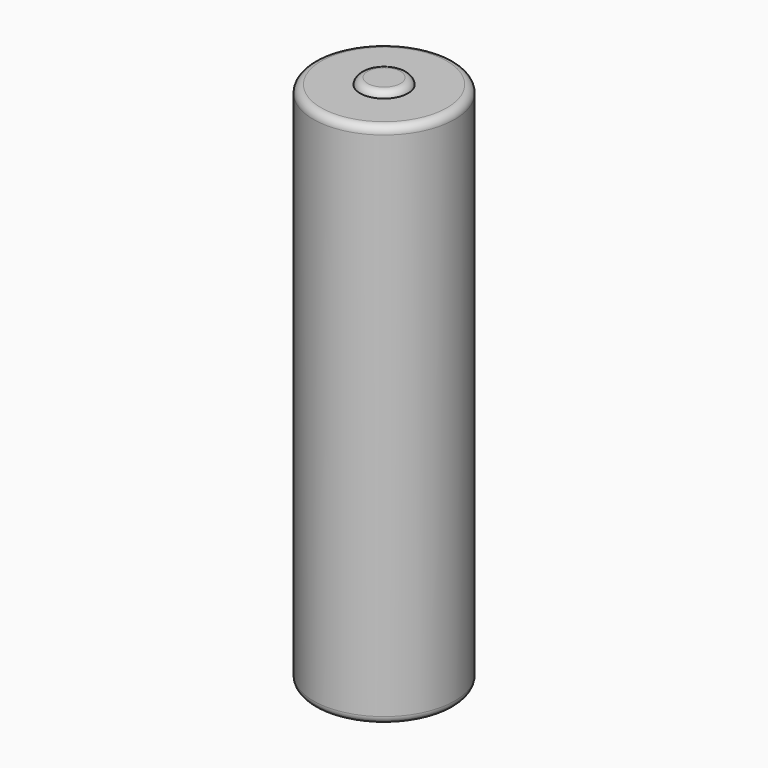
from build123d import *

# Parameters (mm, degrees)
F0_R     = 9.15
F0_R_2   = 3.1
F1_DEPTH = 68.2
F2_DEPTH = 69


# Not quite as in the source:
# - a fillet or chamfer that OpenCascade refuses, or shapes differently, is made with other operations: its cross-section is extruded or revolved along the edge and cut away or added


with BuildPart() as f1:
    # F0 (on Top) → F1 (new body)
    with BuildSketch(Plane.XY):
        Circle(F0_R)
        Circle(F0_R_2, mode=Mode.SUBTRACT)
    extrude(amount=F1_DEPTH)

    # F0 (on Top) → F2 (join)
    with BuildSketch(Plane.XY):
        Circle(F0_R_2)
    extrude(amount=F2_DEPTH)

    # F3: fillet of radius 1 on 3 edges, made by hand

    # F3_s1 → F3_t2 (revolve, cut)
    with BuildSketch(Plane.XZ):
        with BuildLine():
            ThreePointArc((3.1, 68.2), (2.7526596349, 68.7745966692), (2.1202041029, 69))
            Line((2.1202041029, 69), (3.1, 69))
            Line((3.1, 69), (3.1, 68.2))
        make_face()
    revolve(axis=Axis((0, 0, 69), (0, 0, 1)), mode=Mode.SUBTRACT)

    # F3_s3 → F3_t4 (revolve, cut)
    with BuildSketch(Plane.XZ):
        with BuildLine():
            ThreePointArc((9.15, 67.2), (8.8571067812, 67.9071067812), (8.15, 68.2))
            Line((8.15, 68.2), (9.15, 68.2))
            Line((9.15, 68.2), (9.15, 67.2))
        make_face()
    revolve(axis=Axis((0, 0, 68.2), (0, 0, 1)), mode=Mode.SUBTRACT)

    # F3_s5 → F3_t6 (revolve, cut)
    with BuildSketch(Plane.XZ):
        with BuildLine():
            ThreePointArc((9.15, 1), (8.8571067812, 0.2928932188), (8.15, 0))
            Line((8.15, 0), (9.15, 0))
            Line((9.15, 0), (9.15, 1))
        make_face()
    revolve(axis=Axis((0, 0, 0), (0, 0, 1)), mode=Mode.SUBTRACT)


solid = f1.part
